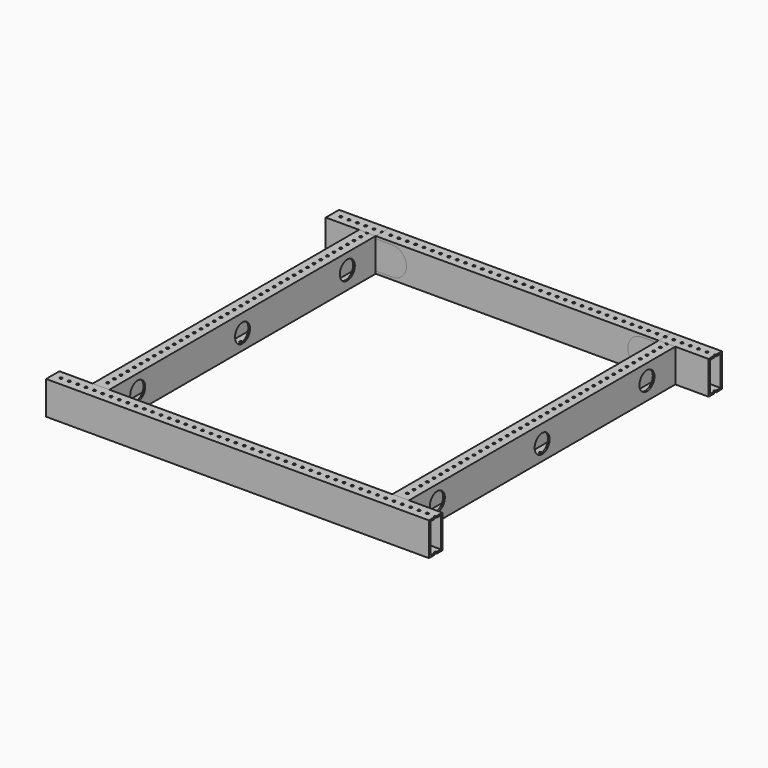
from build123d import *

# Parameters (mm, degrees)
F0_W           = 25.4
F0_H           = 50.8
F0_W_2         = 20.32
F0_H_2         = 45.72
F1_DEPTH       = 292.1
F2_R           = 1.984375
F3_DEPTH       = 76.2
F5_ANGLE       = 270
F7_W           = 25.4
F7_H           = 50.8
F7_W_2         = 20.32
F7_H_2         = 45.72
F8_DEPTH       = 508
F9_R           = 1.984375
F10_DEPTH      = 76.2
F11_R          = 14.2875
F12_DEPTH      = 762
F14_W          = 25.4
F14_H          = 50.8
F14_W_2        = 20.32
F14_H_2        = 45.72
F15_DEPTH      = 215.9
F15_DEPTH_BACK = 215.9
F16_R          = 2.38125
F17_DEPTH      = 50.801
F18_W          = 25.4
F18_H          = 43.18
F19_DEPTH      = 27.94


with BuildPart() as f1:
    # F0 (on Right) → F1 (new body, symmetric)
    with BuildSketch(Plane.YZ):
        Rectangle(F0_W, F0_H)
        Rectangle(F0_W_2, F0_H_2, mode=Mode.SUBTRACT)
    extrude(amount=F1_DEPTH, both=True)

    # F2 (on face) → F3 (cut)
    with BuildSketch(Plane.XY.offset(25.4)):
        with Locations((-279.4, 0)):
            Circle(F2_R)
        with Locations((-266.7, 0)):
            Circle(F2_R)
        with Locations((-254, 0)):
            Circle(F2_R)
        with Locations((-241.3, 0)):
            Circle(F2_R)
        with Locations((-228.6, 0)):
            Circle(F2_R)
        with Locations((-215.9, 0)):
            Circle(F2_R)
        with Locations((-203.2, 0)):
            Circle(F2_R)
        with Locations((-190.5, 0)):
            Circle(F2_R)
        with Locations((-177.8, 0)):
            Circle(F2_R)
        with Locations((-165.1, 0)):
            Circle(F2_R)
        with Locations((-152.4, 0)):
            Circle(F2_R)
        with Locations((-139.7, 0)):
            Circle(F2_R)
        with Locations((-127, 0)):
            Circle(F2_R)
        with Locations((-114.3, 0)):
            Circle(F2_R)
        with Locations((-101.6, 0)):
            Circle(F2_R)
        with Locations((-88.9, 0)):
            Circle(F2_R)
        with Locations((-76.2, 0)):
            Circle(F2_R)
        with Locations((-63.5, 0)):
            Circle(F2_R)
        with Locations((-50.8, 0)):
            Circle(F2_R)
        with Locations((-38.1, 0)):
            Circle(F2_R)
        with Locations((-25.4, 0)):
            Circle(F2_R)
        with Locations((-12.7, 0)):
            Circle(F2_R)
        Circle(F2_R)
        with Locations((12.7, 0)):
            Circle(F2_R)
        with Locations((25.4, 0)):
            Circle(F2_R)
        with Locations((38.1, 0)):
            Circle(F2_R)
        with Locations((50.8, 0)):
            Circle(F2_R)
        with Locations((63.5, 0)):
            Circle(F2_R)
        with Locations((76.2, 0)):
            Circle(F2_R)
        with Locations((88.9, 0)):
            Circle(F2_R)
        with Locations((101.6, 0)):
            Circle(F2_R)
        with Locations((114.3, 0)):
            Circle(F2_R)
        with Locations((127, 0)):
            Circle(F2_R)
        with Locations((139.7, 0)):
            Circle(F2_R)
        with Locations((152.4, 0)):
            Circle(F2_R)
        with Locations((165.1, 0)):
            Circle(F2_R)
        with Locations((177.8, 0)):
            Circle(F2_R)
        with Locations((190.5, 0)):
            Circle(F2_R)
        with Locations((203.2, 0)):
            Circle(F2_R)
        with Locations((215.9, 0)):
            Circle(F2_R)
        with Locations((228.6, 0)):
            Circle(F2_R)
        with Locations((241.3, 0)):
            Circle(F2_R)
        with Locations((254, 0)):
            Circle(F2_R)
        with Locations((266.7, 0)):
            Circle(F2_R)
        with Locations((279.4, 0)):
            Circle(F2_R)
        with Locations((292.1, 0)):
            Circle(F2_R)
        with Locations((304.8, 0)):
            Circle(F2_R)
        with Locations((317.5, 0)):
            Circle(F2_R)
        with Locations((330.2, 0)):
            Circle(F2_R)
        with Locations((342.9, 0)):
            Circle(F2_R)
        with Locations((355.6, 0)):
            Circle(F2_R)
        with Locations((368.3, 0)):
            Circle(F2_R)
        with Locations((381, 0)):
            Circle(F2_R)
        with Locations((393.7, 0)):
            Circle(F2_R)
        with Locations((406.4, 0)):
            Circle(F2_R)
        with Locations((419.1, 0)):
            Circle(F2_R)
        with Locations((431.8, 0)):
            Circle(F2_R)
        with Locations((444.5, 0)):
            Circle(F2_R)
        with Locations((457.2, 0)):
            Circle(F2_R)
        with Locations((469.9, 0)):
            Circle(F2_R)
    extrude(amount=-F3_DEPTH, mode=Mode.SUBTRACT)


with BuildPart() as f4_1:
    # F4: copy of F1
    add(f1.part.moved(Location((0, -533.4, 0))))


with BuildPart() as f5_1:
    # F5: copy of F1
    add(f1.part.rotate(Axis((-292.1, -12.7, 0), (0, 0, 1)), F5_ANGLE))


with BuildPart() as f8:
    # F7 (on face) → F8 (new body)
    with BuildSketch(Plane.XZ.offset(12.7)):
        with Locations((-228.6, 0)):
            Rectangle(F7_W, F7_H)
        with Locations((-228.6, 0)):
            Rectangle(F7_W_2, F7_H_2, mode=Mode.SUBTRACT)
    extrude(amount=F8_DEPTH)

    # F9 (on face) → F10 (cut)
    with BuildSketch(Plane.XY.offset(25.4)):
        with Locations((-228.6, -12.7)):
            Circle(F9_R)
        with Locations((-228.6, -25.4)):
            Circle(F9_R)
        with Locations((-228.6, -38.1)):
            Circle(F9_R)
        with Locations((-228.6, -50.8)):
            Circle(F9_R)
        with Locations((-228.6, -63.5)):
            Circle(F9_R)
        with Locations((-228.6, -76.2)):
            Circle(F9_R)
        with Locations((-228.6, -88.9)):
            Circle(F9_R)
        with Locations((-228.6, -101.6)):
            Circle(F9_R)
        with Locations((-228.6, -114.3)):
            Circle(F9_R)
        with Locations((-228.6, -127)):
            Circle(F9_R)
        with Locations((-228.6, -139.7)):
            Circle(F9_R)
        with Locations((-228.6, -152.4)):
            Circle(F9_R)
        with Locations((-228.6, -165.1)):
            Circle(F9_R)
        with Locations((-228.6, -177.8)):
            Circle(F9_R)
        with Locations((-228.6, -190.5)):
            Circle(F9_R)
        with Locations((-228.6, -203.2)):
            Circle(F9_R)
        with Locations((-228.6, -215.9)):
            Circle(F9_R)
        with Locations((-228.6, -228.6)):
            Circle(F9_R)
        with Locations((-228.6, -241.3)):
            Circle(F9_R)
        with Locations((-228.6, -254)):
            Circle(F9_R)
        with Locations((-228.6, -266.7)):
            Circle(F9_R)
        with Locations((-228.6, -279.4)):
            Circle(F9_R)
        with Locations((-228.6, -292.1)):
            Circle(F9_R)
        with Locations((-228.6, -304.8)):
            Circle(F9_R)
        with Locations((-228.6, -317.5)):
            Circle(F9_R)
        with Locations((-228.6, -330.2)):
            Circle(F9_R)
        with Locations((-228.6, -342.9)):
            Circle(F9_R)
        with Locations((-228.6, -355.6)):
            Circle(F9_R)
        with Locations((-228.6, -368.3)):
            Circle(F9_R)
        with Locations((-228.6, -381)):
            Circle(F9_R)
        with Locations((-228.6, -393.7)):
            Circle(F9_R)
        with Locations((-228.6, -406.4)):
            Circle(F9_R)
        with Locations((-228.6, -419.1)):
            Circle(F9_R)
        with Locations((-228.6, -431.8)):
            Circle(F9_R)
        with Locations((-228.6, -444.5)):
            Circle(F9_R)
        with Locations((-228.6, -457.2)):
            Circle(F9_R)
        with Locations((-228.6, -469.9)):
            Circle(F9_R)
        with Locations((-228.6, -482.6)):
            Circle(F9_R)
        with Locations((-228.6, -495.3)):
            Circle(F9_R)
        with Locations((-228.6, -508)):
            Circle(F9_R)
    extrude(amount=-F10_DEPTH, mode=Mode.SUBTRACT)

    # F11 (on face) → F12 (cut, symmetric)
    with BuildSketch(Plane(origin=(-241.3, 0, 0), x_dir=(0, -1, 0), z_dir=(-1, 0, 0))):
        with Locations((266.7, -1.5875)):
            Circle(F11_R)
        with Locations((466.6069546099, 1.5875)):
            Circle(F11_R)
        with Locations((66.7930453901, 1.5875)):
            Circle(F11_R)
    extrude(amount=F12_DEPTH, both=True, mode=Mode.SUBTRACT)


with BuildPart() as f13_1:
    # F13: instance of F8
    add(f8.part.mirror(Plane.YZ))


with BuildPart() as f15:
    # F14 (on Right) → F15 (new body, two sides)
    with BuildSketch(Plane.YZ) as f15_sk:
        Rectangle(F14_W, F14_H)
        Rectangle(F14_W_2, F14_H_2, mode=Mode.SUBTRACT)
    extrude(amount=-F15_DEPTH)
    extrude(f15_sk.sketch, amount=F15_DEPTH_BACK)

    # F16 (on face) → F17 (cut, through all)
    with BuildSketch(Plane.XY.offset(25.4)):
        with Locations((-203.2, 0)):
            Circle(F16_R)
        with Locations((-190.5, 0)):
            Circle(F16_R)
        with Locations((-177.8, 0)):
            Circle(F16_R)
        with Locations((-165.1, 0)):
            Circle(F16_R)
        with Locations((-152.4, 0)):
            Circle(F16_R)
        with Locations((-139.7, 0)):
            Circle(F16_R)
        with Locations((-127, 0)):
            Circle(F16_R)
        with Locations((-114.3, 0)):
            Circle(F16_R)
        with Locations((-101.6, 0)):
            Circle(F16_R)
        with Locations((-88.9, 0)):
            Circle(F16_R)
        with Locations((-76.2, 0)):
            Circle(F16_R)
        with Locations((-63.5, 0)):
            Circle(F16_R)
        with Locations((-50.8, 0)):
            Circle(F16_R)
        with Locations((-38.1, 0)):
            Circle(F16_R)
        with Locations((-25.4, 0)):
            Circle(F16_R)
        with Locations((-12.7, 0)):
            Circle(F16_R)
        Circle(F16_R)
        with Locations((12.7, 0)):
            Circle(F16_R)
        with Locations((25.4, 0)):
            Circle(F16_R)
        with Locations((38.1, 0)):
            Circle(F16_R)
        with Locations((50.8, 0)):
            Circle(F16_R)
        with Locations((63.5, 0)):
            Circle(F16_R)
        with Locations((76.2, 0)):
            Circle(F16_R)
        with Locations((88.9, 0)):
            Circle(F16_R)
        with Locations((101.6, 0)):
            Circle(F16_R)
        with Locations((114.3, 0)):
            Circle(F16_R)
        with Locations((127, 0)):
            Circle(F16_R)
        with Locations((139.7, 0)):
            Circle(F16_R)
        with Locations((152.4, 0)):
            Circle(F16_R)
        with Locations((165.1, 0)):
            Circle(F16_R)
        with Locations((177.8, 0)):
            Circle(F16_R)
        with Locations((190.5, 0)):
            Circle(F16_R)
        with Locations((203.2, 0)):
            Circle(F16_R)
        with Locations((215.9, 0)):
            Circle(F16_R)
        with Locations((228.6, 0)):
            Circle(F16_R)
        with Locations((241.3, 0)):
            Circle(F16_R)
        with Locations((254, 0)):
            Circle(F16_R)
        with Locations((266.7, 0)):
            Circle(F16_R)
        with Locations((279.4, 0)):
            Circle(F16_R)
        with Locations((292.1, 0)):
            Circle(F16_R)
    extrude(amount=-F17_DEPTH, mode=Mode.SUBTRACT)

    # F18 (on face) → F19 (cut)
    with BuildSketch(Plane.XZ.offset(12.7)):
        with Locations((-203.2, 0)):
            Rectangle(F18_W, F18_H)
        with BuildLine():
            ThreePointArc((-190.5, -21.59), (-168.91, 0), (-190.5, 21.59))
            Line((-190.5, 21.59), (-190.5, -21.59))
        make_face()
        with BuildLine():
            Line((190.5, -21.59), (190.5, 21.59))
            ThreePointArc((190.5, 21.59), (168.91, 0), (190.5, -21.59))
        make_face()
        with Locations((203.2, 0)):
            Rectangle(F18_W, F18_H)
    extrude(amount=-F19_DEPTH, mode=Mode.SUBTRACT)


solid = Compound([f1.part, f4_1.part, f8.part, f13_1.part, f15.part])
